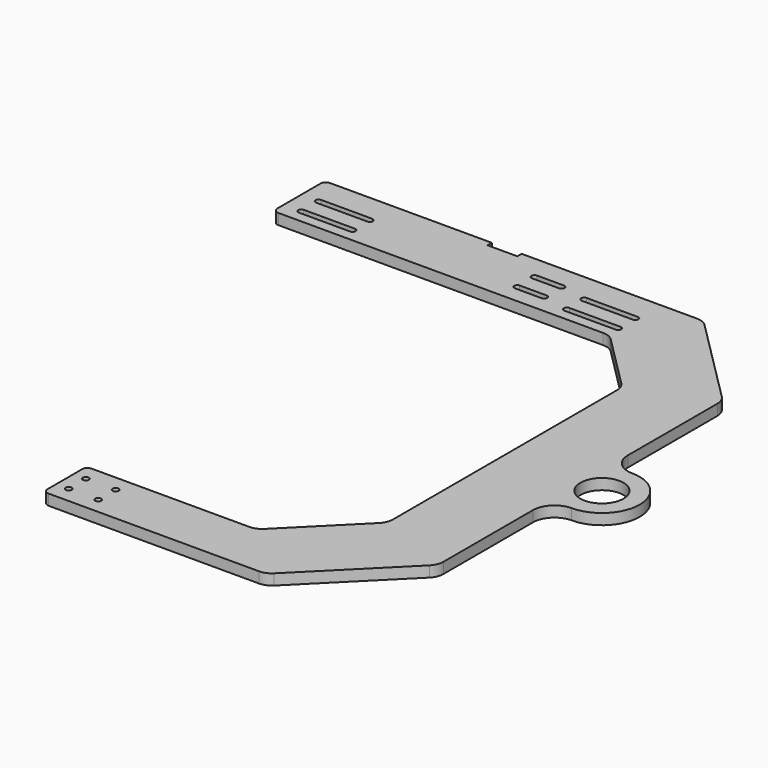
from build123d import *

# Parameters (mm, degrees)
F0_R     = 3.5687
F0_R_2   = 25.4
F1_DEPTH = 12.7
F2_R     = 25.39999
F3_R     = 19.05
F4_R     = 6.35


# Not quite as in the source:
# - a fillet or chamfer is up to 0.001 mm smaller than in the source, because OpenCascade refuses the exact size


with BuildPart() as f1:
    # F0 (on Top) → F1 (new body)
    with BuildSketch(Plane.XY):
        with BuildLine():
            Line((-25.4, -44.45), (0, -44.45))
            ThreePointArc((0, -44.45), (44.45, 0), (0, 44.45))
            Line((0, 44.45), (-25.4, 44.45))
            Line((-25.4, 44.45), (-25.4, 209.55))
            Line((-25.4, 209.55), (-138.1252, 322.2752))
            Line((-138.1252, 322.2752), (-352.425, 322.2752))
            Line((-352.425, 322.2752), (-352.425, 315.9252107143))
            Line((-352.425, 315.9252107143), (-387.35, 315.9252107143))
            Line((-387.35, 315.9252107143), (-387.35, 322.2752))
            Line((-387.35, 322.2752), (-584.2, 322.2752))
            Line((-584.2, 322.2752), (-584.2, 246.0752))
            Line((-584.2, 246.0752), (-187.648785695, 246.0752))
            Line((-187.648785695, 246.0752), (-114.3, 172.726414305))
            Line((-114.3, 172.726414305), (-114.3, -172.726414305))
            Line((-114.3, -172.726414305), (-200.348785695, -258.7752))
            Line((-200.348785695, -258.7752), (-400.05, -258.7752))
            Line((-400.05, -258.7752), (-400.05, -322.2752))
            Line((-400.05, -322.2752), (-138.1252, -322.2752))
            Line((-138.1252, -322.2752), (-25.4, -209.55))
            Line((-25.4, -209.55), (-25.4, -44.45))
        make_face()
        with Locations((-385.3688, -303.2252)):
            Circle(F0_R, mode=Mode.SUBTRACT)
        with Locations((-350.4438, -303.2252)):
            Circle(F0_R, mode=Mode.SUBTRACT)
        with Locations((-385.3688, -277.8252)):
            Circle(F0_R, mode=Mode.SUBTRACT)
        with Locations((-350.4438, -277.8252)):
            Circle(F0_R, mode=Mode.SUBTRACT)
        with BuildLine():
            Line((-503.2502, 258.3815), (-563.5752, 258.3815))
            ThreePointArc((-563.5752, 258.3815), (-567.1439, 261.9502), (-563.5752, 265.5189))
            Line((-563.5752, 265.5189), (-503.2502, 265.5189))
            ThreePointArc((-503.2502, 265.5189), (-499.6815, 261.9502), (-503.2502, 258.3815))
        make_face(mode=Mode.SUBTRACT)
        with BuildLine():
            ThreePointArc((-563.5752, 283.7815), (-567.1439, 287.3502), (-563.5752, 290.9189))
            Line((-563.5752, 290.9189), (-503.2502, 290.9189))
            ThreePointArc((-503.2502, 290.9189), (-499.6815, 287.3502), (-503.2502, 283.7815))
            Line((-503.2502, 283.7815), (-563.5752, 283.7815))
        make_face(mode=Mode.SUBTRACT)
        with BuildLine():
            Line((-282.575, 264.7315), (-314.325, 264.7315))
            ThreePointArc((-314.325, 264.7315), (-317.8937, 268.3002), (-314.325, 271.8689))
            Line((-314.325, 271.8689), (-282.575, 271.8689))
            ThreePointArc((-282.575, 271.8689), (-279.0063, 268.3002), (-282.575, 264.7315))
        make_face(mode=Mode.SUBTRACT)
        with BuildLine():
            Line((-282.575, 290.1315), (-314.325, 290.1315))
            ThreePointArc((-314.325, 290.1315), (-317.8937, 293.7002), (-314.325, 297.2689))
            Line((-314.325, 297.2689), (-282.575, 297.2689))
            ThreePointArc((-282.575, 297.2689), (-279.0063, 293.7002), (-282.575, 290.1315))
        make_face(mode=Mode.SUBTRACT)
        Circle(F0_R_2, mode=Mode.SUBTRACT)
        with BuildLine():
            Line((-190.5, 258.3815), (-250.825, 258.3815))
            ThreePointArc((-250.825, 258.3815), (-254.3937, 261.9502), (-250.825, 265.5189))
            Line((-250.825, 265.5189), (-190.5, 265.5189))
            ThreePointArc((-190.5, 265.5189), (-186.9313, 261.9502), (-190.5, 258.3815))
        make_face(mode=Mode.SUBTRACT)
        with BuildLine():
            ThreePointArc((-250.825, 283.7815), (-254.3937, 287.3502), (-250.825, 290.9189))
            Line((-250.825, 290.9189), (-190.5, 290.9189))
            ThreePointArc((-190.5, 290.9189), (-186.9313, 287.3502), (-190.5, 283.7815))
            Line((-190.5, 283.7815), (-250.825, 283.7815))
        make_face(mode=Mode.SUBTRACT)
    extrude(amount=F1_DEPTH)

    # F2 (radius 25.4 in the source; OpenCascade refuses exactly that, so slightly less here)
    f2_edges = [f1.edges().sort_by_distance(p)[0] for p in [
        (-25.4, -44.45, 6.35),
        (-25.4, 44.45, 6.35),
    ]]
    fillet(f2_edges, radius=F2_R)

    # F3
    f3_edges = [f1.edges().sort_by_distance(p)[0] for p in [
        (-25.4, -209.55, 6.35),
        (-138.1252, -322.2752, 6.35),
        (-25.4, 209.55, 6.35),
        (-138.1252, 322.2752, 6.35),
        (-114.3, 172.726414, 6.35),
        (-187.648786, 246.0752, 6.35),
        (-114.3, -172.726414, 6.35),
        (-200.348786, -258.7752, 6.35),
    ]]
    fillet(f3_edges, radius=F3_R)

    # F4
    f4_edges = [f1.edges().sort_by_distance(p)[0] for p in [
        (-400.05, -258.7752, 6.35),
        (-400.05, -322.2752, 6.35),
        (-584.2, 246.0752, 6.35),
        (-584.2, 322.2752, 6.35),
    ]]
    fillet(f4_edges, radius=F4_R)


solid = f1.part
